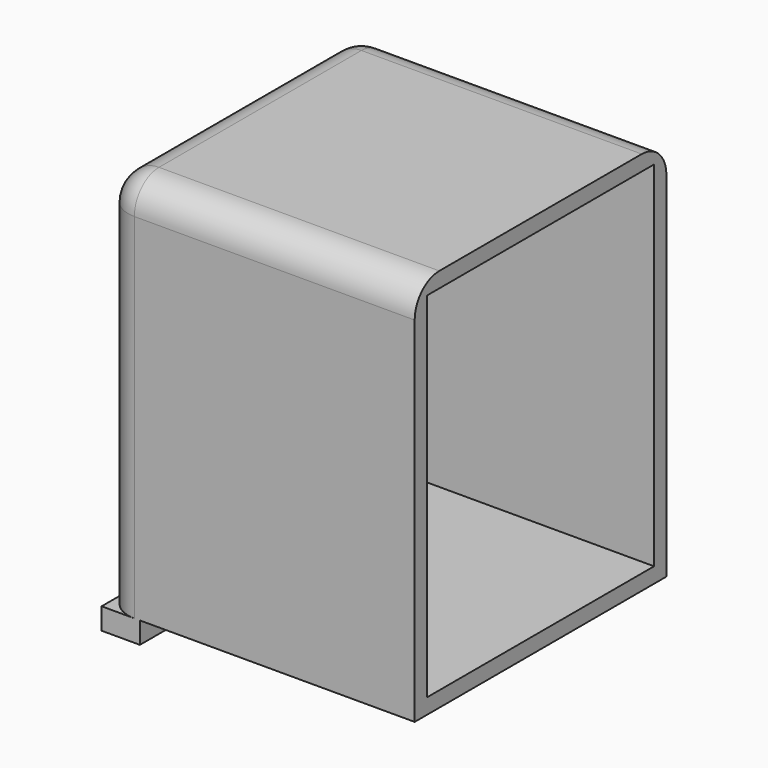
from build123d import *

# Parameters (mm, degrees)
F0_W         = 51.3733290136
F0_H         = 51.9489385188
F1_DEPTH     = 63.5
F3_DEPTH     = 3.556
F4_T         = 2.54
F4_T3_DEPTH  = 13.7734491992
F4_T5_DEPTH  = 11.8834199066
F4_T7_DEPTH  = 11.0801313686
F4_T9_DEPTH  = 13.5809922736
F4_T11_DEPTH = 10.8262574938
F4_T13_DEPTH = 5.3370977176
F5_T1_DEPTH  = 76.2
F6_R         = 5.08


# Not quite as in the source:
# - a fillet or chamfer that OpenCascade refuses, or shapes differently, is made with other operations: its cross-section is extruded or revolved along the edge and cut away or added
# - a shell that OpenCascade refuses in one call is made with other operations: the cavity is built on its own and cut out


with BuildPart() as f1:
    # F0 (on Top) → F1 (new body)
    with BuildSketch(Plane.XY):
        with Locations((-25.6866645068, 25.9744692594)):
            Rectangle(F0_W, F0_H)
    extrude(amount=F1_DEPTH)

    # F2 (on Top) → F3 (join)
    with BuildSketch(Plane.XY):
        Polygon((-51.6957342625, 3.4017099533), (-51.6957342625, 0), (-45.3731976449, 0), (-45.3731976449, 6.8034199066), (-51.6957342625, 6.8034199066), align=None)
        Polygon((-45.3731976449, 43.2554893196), (-45.3731976449, 51.7564815932), (-51.6957342625, 51.9683584571), (-51.6957342625, 47.6119238883), (-51.6957342625, 43.2554893196), align=None)
    extrude(amount=-F3_DEPTH)

    # F4: shell of thickness 2.54, made by hand


with BuildPart() as f4_core1:
    # F4_t2: copy of F1
    add(f1.part)

    # the walls: a layer under each face that stays
    f4_faces = [f4_core1.faces().sort_by_distance(p)[0] for p in [
        (-25.8478671312, 0, 29.972),
        (-51.3733290136, 25.9744692594, 31.75),
        (-25.6866645068, 25.9744692594, 0),
        (-25.6866645068, 25.9744692594, 63.5),
        (-25.6866645068, 51.9489385188, 31.75),
        (-51.4059827792, 47.6119238883, 0),
        (-51.534531638, 3.4017099533, 0),
        (-51.6957342625, 3.4017099533, -1.778),
        (-45.3731976449, 3.4017099533, -1.778),
        (-48.5344659537, 3.4017099533, -3.556),
        (-48.5344659537, 6.8034199066, -1.778),
        (-48.5344659537, 43.2554893196, -1.778),
        (-45.3731976449, 47.5059854564, -1.778),
        (-48.5344659537, 51.8624200251, -1.778),
        (-51.6957342625, 47.6119238883, -1.778),
        (-48.5344659537, 47.6119238883, -3.556),
    ]]
    thicken(f4_faces, amount=-F4_T, mode=Mode.SUBTRACT)

    # F4_s4 → F4_t3 (cut)
    with BuildSketch(Plane.XZ.offset(-54.4889385188)):
        Polygon((-51.3987290136, 0.0254), (-48.8333290136, 0), (-48.8333290136, -2.54), (-51.3733290136, -2.54), align=None)
    extrude(amount=F4_T3_DEPTH, mode=Mode.SUBTRACT)

    # F4_s6 → F4_t5 (cut)
    with BuildSketch(Plane.XZ.offset(-9.3434199066)):
        Polygon((-51.3987290136, 0.0254), (-48.8333290136, 0), (-48.8333290136, -2.54), (-51.3733290136, -2.54), align=None)
        Polygon((-45.3477976449, -0.0254), (-45.3731976449, 2.54), (-47.9131976449, 2.54), (-47.9131976449, 0), align=None)
    extrude(amount=F4_T5_DEPTH, mode=Mode.SUBTRACT)

    # F4_s8 → F4_t7 (cut)
    with BuildSketch(Plane.YZ.offset(-53.9133290136)):
        Polygon((6.8288199066, -0.0254), (6.8034199066, 2.54), (4.2634199066, 2.54), (4.2634199066, 0), align=None)
        Polygon((43.2300893196, -0.0254), (43.2554893196, 2.54), (45.7954893196, 2.54), (45.7954893196, 0), align=None)
    extrude(amount=F4_T7_DEPTH, mode=Mode.SUBTRACT)

    # F4_s10 → F4_t9 (cut)
    with BuildSketch(Plane.XZ.offset(-54.2964815932)):
        Polygon((-45.3477976449, -0.0254), (-45.3731976449, 2.54), (-47.9131976449, 2.54), (-47.9131976449, 0), align=None)
    extrude(amount=F4_T9_DEPTH, mode=Mode.SUBTRACT)

    # F4_s12 → F4_t11 (cut)
    with BuildSketch(Plane(origin=(-44.5162101899, 1.4917991907, 0), x_dir=(0, 0, 1), z_dir=(-0.9994389665, 0.033492569, 0))):
        Polygon((-0.0254, 50.2331795219), (2.54, 50.2077795219), (2.54, 47.6677795219), (0, 47.6677795219), align=None)
    extrude(amount=F4_T11_DEPTH, mode=Mode.SUBTRACT)

    # F4_s14 → F4_t13 (cut)
    with BuildSketch(Plane.YZ.offset(-53.9133290136)):
        Polygon((51.9743385188, 0.0254), (49.4089385188, 0), (49.4089385188, -2.54), (51.9489385188, -2.54), align=None)
    extrude(amount=F4_T13_DEPTH, mode=Mode.SUBTRACT)


with BuildPart() as f1_1:
    add(f1.part)

    # what is left inside the walls is the cavity
    f4_cavity = [f4_core1.part.solids().sort_by_distance(p)[0] for p in [
        (-24.416665, 2.5654, 40.301333),
    ]]
    add(f4_cavity, mode=Mode.SUBTRACT)

    # F5: fillet of radius 5.08 on 2 edges, made by hand

    # F5_s2 → F5_t1 (cut)
    with BuildSketch(Plane.XY):
        with BuildLine():
            ThreePointArc((-46.2933290136, 0), (-49.885431462, 1.4878975516), (-51.3733290136, 5.08))
            Line((-51.3733290136, 5.08), (-51.3733290136, 0))
            Line((-51.3733290136, 0), (-46.2933290136, 0))
        make_face()
        with BuildLine():
            ThreePointArc((-51.3733290136, 46.8689385188), (-49.885431462, 50.4610409672), (-46.2933290136, 51.9489385188))
            Line((-46.2933290136, 51.9489385188), (-51.3733290136, 51.9489385188))
            Line((-51.3733290136, 51.9489385188), (-51.3733290136, 46.8689385188))
        make_face()
    extrude(amount=F5_T1_DEPTH, mode=Mode.SUBTRACT)

    # F6
    f6_edges = [f1_1.edges().sort_by_distance(p)[0] for p in [
        (-51.373329, 25.974469, 63.5),
        (-23.146665, 0, 63.5),
        (-23.146665, 51.948939, 63.5),
        (-49.885431, 50.461041, 63.5),
        (-49.885431, 1.487898, 63.5),
    ]]
    fillet(f6_edges, radius=F6_R)


solid = f1_1.part
